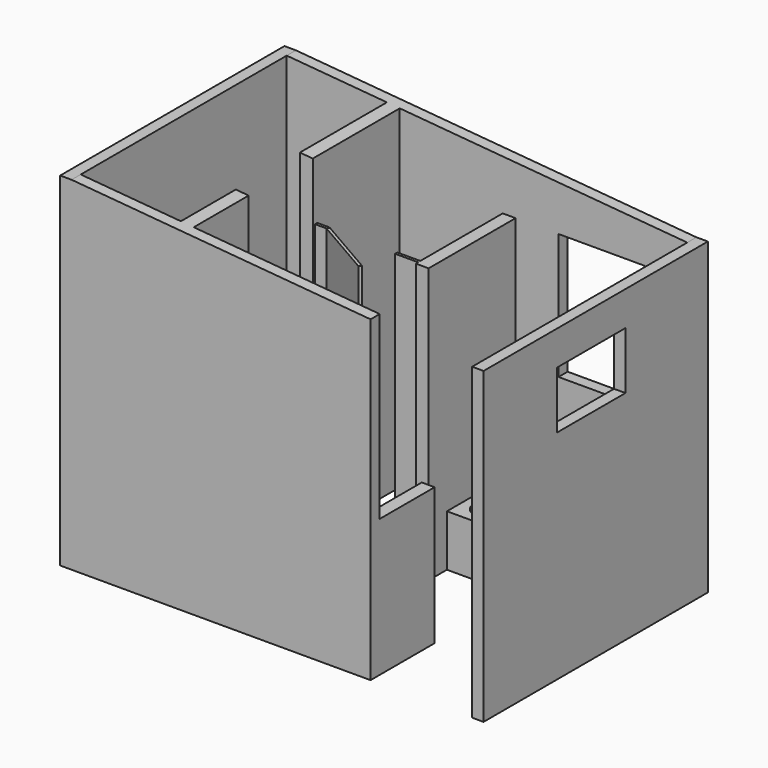
from build123d import *

# Parameters (mm, degrees)
F2_DEPTH      = 3048
F1_W          = 114.3
F1_H          = 965.2
F1_H_2        = 609.6
F3_DEPTH      = 3048
F4_DEPTH      = 2438.4
F5_W          = 101.6
F5_H          = 304.8
F6_DEPTH      = 2387.601
F6_DEPTH_BACK = 101.601
F7_W          = 1524
F7_H          = 762
F8_DEPTH      = 457.2
F9_T          = -76.2
F10_R         = 127
F12_DEPTH     = 2438.4
F11_W         = 203.2
F11_H         = 25.4
F13_DEPTH     = 2438.4
F11_W_2       = 101.6
F14_W         = 762
F14_H         = 1117.6
F15_DEPTH     = 101.601
F16_W         = 1524
F16_H         = 508
F17_DEPTH     = 914.4
F18_W         = 304.8
F18_H         = 203.2
F19_DEPTH     = 203.2
F20_R         = 50.8
F22_DEPTH     = 508
F23_DEPTH     = 711.2
F24_W         = 889
F24_H         = 609.6
F25_DEPTH     = 2438.4
F26_W         = 762
F26_H         = 508
F27_DEPTH     = 101.601
F28_DEPTH     = 1219.2


with BuildPart() as f2:
    # F0 (on Top) → F2 (new body)
    with BuildSketch(Plane.XY):
        Polygon((-3556, 0), (-3556, 2286), (0, 2286), (0, -101.6), (101.6, -101.6), (101.6, 2387.6), (-3657.6, 2387.6), (-3657.6, -101.6), (-901.7, -101.6), (-901.7, 0), align=None)
    extrude(amount=F2_DEPTH)

    # F1 (on Top) → F3 (join, through all)
    with BuildSketch(Plane.XY):
        with Locations((-2609.85, 1803.4)):
            Rectangle(F1_W, F1_H)
        with Locations((-2609.85, 304.8)):
            Rectangle(F1_W, F1_H_2)
    extrude(amount=F3_DEPTH)

    # F1 (on Top) → F4 (join)
    with BuildSketch(Plane.XY):
        with Locations((-1581.15, 1803.4)):
            Rectangle(F1_W, F1_H)
    extrude(amount=F4_DEPTH)

    # F5 (on Front) → F6 (cut, two sides)
    with BuildSketch(Plane.XZ) as f6_sk:
        Polygon((0, 3048), (-3556, 3048), (0, 2743.2), align=None)
        with Locations((50.8, 2895.6)):
            Rectangle(F5_W, F5_H)
    extrude(amount=-F6_DEPTH, mode=Mode.SUBTRACT)
    extrude(f6_sk.sketch, amount=F6_DEPTH_BACK, mode=Mode.SUBTRACT)

    # F14 (on face) → F15 (cut, through all)
    with BuildSketch(Plane.XZ.offset(-2286)):
        with Locations((-762, 1879.6)):
            Rectangle(F14_W, F14_H)
    extrude(amount=-F15_DEPTH, mode=Mode.SUBTRACT)

    # F26 (on face) → F27 (cut, through all)
    with BuildSketch(Plane(origin=(0, 0, 0), x_dir=(0, -1, 0), z_dir=(-1, 0, 0))):
        with Locations((-1092.2, 2184.4)):
            Rectangle(F26_W, F26_H)
    extrude(amount=-F27_DEPTH, mode=Mode.SUBTRACT)

    # F1 (on Top) → F28 (join)
    with BuildSketch(Plane.XY):
        with Locations((-958.85, 304.8)):
            Rectangle(F1_W, F1_H_2)
    extrude(amount=F28_DEPTH)


with BuildPart() as f8:
    # F7 (on Top) → F8 (new body)
    with BuildSketch(Plane.XY):
        with Locations((-762, 1905)):
            Rectangle(F7_W, F7_H)
    extrude(amount=F8_DEPTH)

    # F9
    f9_openings = [f8.faces().sort_by_distance(p)[0] for p in [
        (-762, 1905, 457.2),
    ]]
    offset(amount=F9_T, openings=f9_openings)

    # F10
    f10_edges = [f8.edges().sort_by_distance(p)[0] for p in [
        (-1447.8, 1600.2, 266.7),
        (-76.2, 1600.2, 266.7),
        (-1447.8, 1905, 76.2),
        (-762, 1600.2, 76.2),
        (-76.2, 1905, 76.2),
        (-762, 2209.8, 76.2),
        (-76.2, 2209.8, 266.7),
        (-1447.8, 2209.8, 266.7),
    ]]
    fillet(f10_edges, radius=F10_R)


with BuildPart() as f12:
    # F11 (on Top) → F12 (new body, through all)
    with BuildSketch(Plane.XY):
        Polygon((-2451.1, 1346.2), (-1923.170913853, 1041.4), (-1910.470913853, 1063.3970452561), (-2438.4, 1368.1970452561), align=None)
    extrude(amount=F12_DEPTH)


with BuildPart() as f13:
    # F11 (on Top) → F13 (new body, through all)
    with BuildSketch(Plane.XY):
        with Locations((-1739.9, 1358.9)):
            Rectangle(F11_W, F11_H)
    extrude(amount=F13_DEPTH)


with BuildPart() as f13b:
    # F11 (on Top) → F13, piece 2 (new body, through all)
    with BuildSketch(Plane.XY):
        with Locations((-2501.9, 1358.9)):
            Rectangle(F11_W_2, F11_H)
    extrude(amount=F13_DEPTH)


with BuildPart() as f17:
    # F16 (on Top) → F17 (new body)
    with BuildSketch(Plane.XY):
        with Locations((-1784.35, 254)):
            Rectangle(F16_W, F16_H)
    extrude(amount=F17_DEPTH)

    # F18 (on face) → F19 (cut)
    with BuildSketch(Plane.XY.offset(914.4)):
        with Locations((-2165.35, 254)):
            Rectangle(F18_W, F18_H)
        with Locations((-1403.35, 254)):
            Rectangle(F18_W, F18_H)
    extrude(amount=-F19_DEPTH, mode=Mode.SUBTRACT)

    # F20
    f20_edges = [f17.edges().sort_by_distance(p)[0] for p in [
        (-2317.75, 355.6, 812.8),
        (-2012.95, 355.6, 812.8),
        (-2317.75, 152.4, 812.8),
        (-2012.95, 152.4, 812.8),
        (-2012.95, 254, 711.2),
        (-2165.35, 355.6, 711.2),
        (-2317.75, 254, 711.2),
        (-2165.35, 152.4, 711.2),
        (-1250.95, 152.4, 812.8),
        (-1555.75, 152.4, 812.8),
        (-1250.95, 355.6, 812.8),
        (-1555.75, 355.6, 812.8),
        (-1403.35, 355.6, 711.2),
        (-1555.75, 254, 711.2),
        (-1403.35, 152.4, 711.2),
        (-1250.95, 254, 711.2),
    ]]
    fillet(f20_edges, radius=F20_R)


with BuildPart() as f22:
    # F21 (on Top) → F22 (new body)
    with BuildSketch(Plane.XY):
        with BuildLine():
            Line((-2904.9580933959, 1930.4), (-3318.0419066041, 1930.4))
            add(Edge.make_bspline(
                [(-3318.0419066041, 1930.4), (-3472.9483365572, 1422.4), (-3111.5, 1422.4), (-2750.0516634428, 1422.4), (-2904.9580933959, 1930.4)],
                knots=[1.1278852827, 1.1278852827, 1.1278852827, 3.1415926536, 3.1415926536, 5.1553000245, 5.1553000245, 5.1553000245], degree=2, weights=[1, 0.5345224838, 1, 0.5345224838, 1]))
        make_face()
        with BuildLine():
            add(Edge.make_bspline(
                [(-2904.9580933959, 1930.4), (-2966.9206653771, 2133.6), (-3111.5, 2133.6)],
                knots=[5.1553000245, 5.1553000245, 5.1553000245, 6.2831853072, 6.2831853072, 6.2831853072], degree=2, weights=[1, 0.8451542547, 1]))
            add(Edge.make_bspline(
                [(-3111.5, 2133.6), (-3256.0793346229, 2133.6), (-3318.0419066041, 1930.4)],
                knots=[0, 0, 0, 1.1278852827, 1.1278852827, 1.1278852827], degree=2, weights=[1, 0.8451542547, 1]))
            Line((-3318.0419066041, 1930.4), (-2904.9580933959, 1930.4))
        make_face()
    extrude(amount=F22_DEPTH)

    # F21 (on Top) → F23 (join)
    with BuildSketch(Plane.XY):
        with BuildLine():
            add(Edge.make_bspline(
                [(-3111.5, 2133.6), (-3256.0793346229, 2133.6), (-3318.0419066041, 1930.4)],
                knots=[0, 0, 0, 1.1278852827, 1.1278852827, 1.1278852827], degree=2, weights=[1, 0.8451542547, 1]))
            add(Edge.make_bspline(
                [(-2904.9580933959, 1930.4), (-2966.9206653771, 2133.6), (-3111.5, 2133.6)],
                knots=[5.1553000245, 5.1553000245, 5.1553000245, 6.2831853072, 6.2831853072, 6.2831853072], degree=2, weights=[1, 0.8451542547, 1]))
            Line((-2904.9580933959, 1930.4), (-2857.5, 1930.4))
            Line((-2857.5, 1930.4), (-2857.5, 2184.4))
            Line((-2857.5, 2184.4), (-3365.5, 2184.4))
            Line((-3365.5, 2184.4), (-3365.5, 1930.4))
            Line((-3365.5, 1930.4), (-3318.0419066041, 1930.4))
        make_face()
    extrude(amount=F23_DEPTH)


with BuildPart() as f25:
    # F24 (on Top) → F25 (new body)
    with BuildSketch(Plane.XY):
        with Locations((-3111.5, 304.8)):
            Rectangle(F24_W, F24_H)
    extrude(amount=F25_DEPTH)


solid = Compound([f2.part, f8.part, f12.part, f13.part, f13b.part, f17.part, f22.part, f25.part])
